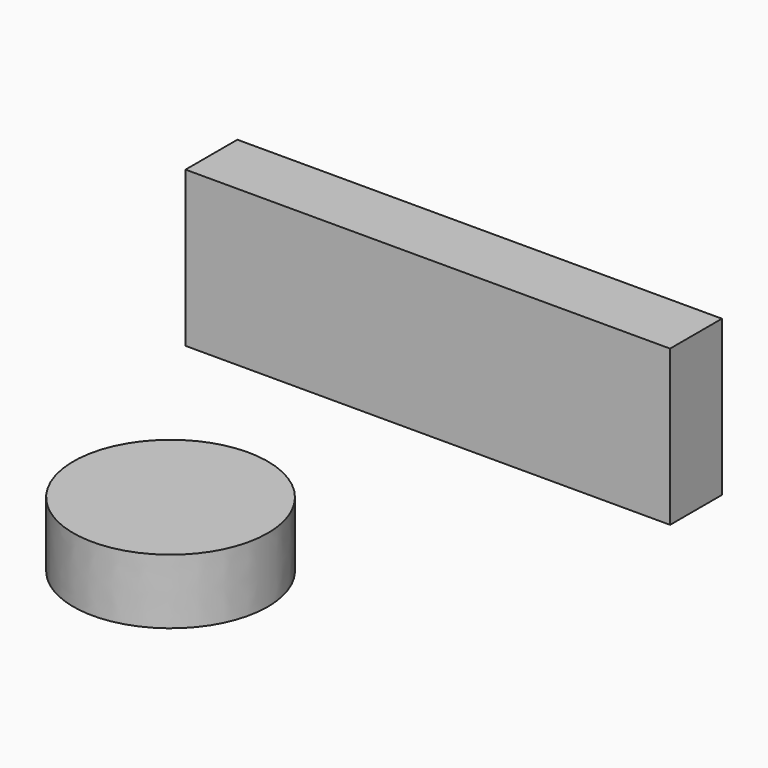
from build123d import *

# Parameters (mm, degrees)
F0_W     = 189.936529845
F0_H     = 60.828410089
F1_DEPTH = 25.4
F5_DEPTH = 25.4


# Not quite as in the source:
# - the program builds the solid bodies; features that only make, move or delete a surface that nothing else refers to are left out


with BuildPart() as f1:
    # F0 (on Front) → F1 (new body)
    with BuildSketch(Plane.XZ):
        with Locations((-69.4125667214, 30.4142050445)):
            Rectangle(F0_W, F0_H)
    extrude(amount=F1_DEPTH)


with BuildPart() as f5:
    # F4 (on face) → F5 (new body)
    with BuildSketch(Plane(origin=(0, 0, 0), x_dir=(1, 0, 0), z_dir=(0, 0, -1))):
        with BuildLine():
            add(Edge.make_bspline(
                [(-67.1733883262, 106.6212207079), (-67.1733883262, 172.6123564763), (-124.3233883262, 139.6167885921), (-181.4733883262, 106.6212207079), (-124.3233883262, 73.6256528237), (-67.1733883262, 40.6300849395), (-67.1733883262, 106.6212207079)],
                knots=[0, 0, 0, 2.0943951024, 2.0943951024, 4.1887902048, 4.1887902048, 6.2831853072, 6.2831853072, 6.2831853072], degree=2, weights=[1, 0.5, 1, 0.5, 1, 0.5, 1]))
        make_face()
    extrude(amount=F5_DEPTH)


solid = Compound([f1.part, f5.part])
